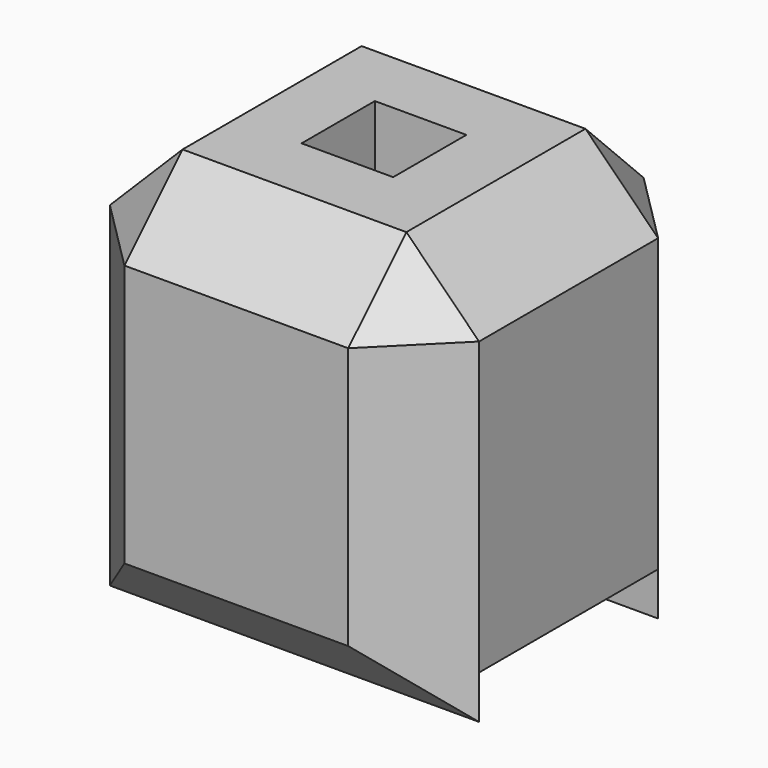
from build123d import *

# Parameters (mm, degrees)
F1_DEPTH = 2.54
F2_SIZE  = 0.49999
F3_W     = 0.63
F3_H     = 0.63
F4_DEPTH = 2.505


# Not quite as in the source:
# - a fillet or chamfer is up to 0.001 mm smaller than in the source, because OpenCascade refuses the exact size


with BuildPart() as f1:
    # F0 (on Right) → F1 (new body)
    with BuildSketch(Plane.YZ):
        Polygon((1.27, 1.402), (-1.27, 1.402), (-1.27, -1.402), (-0.77, -1.402), (-0.77, -1.103), (0.77, -1.103), (0.77, -1.402), (1.27, -1.402), align=None)
    extrude(amount=F1_DEPTH)

    # F2 (size 0.5 in the source; OpenCascade refuses exactly that, so slightly less here)
    f2_edges = [f1.edges().sort_by_distance(p)[0] for p in [
        (2.54, 0, 1.402),
        (0, 0, 1.402),
        (1.27, -1.27, 1.402),
        (1.27, 1.27, 1.402),
        (2.54, 1.27, 0),
        (1.27, 1.27, -1.402),
        (0, 1.27, 0),
        (2.54, -1.27, 0),
        (0, -1.27, 0),
        (1.27, -1.27, -1.402),
    ]]
    chamfer(f2_edges, length=F2_SIZE)

    # F3 (on face) → F4 (cut, through all)
    with BuildSketch(Plane.XY.offset(1.402)):
        with Locations((1.27, 0)):
            Rectangle(F3_W, F3_H)
    extrude(amount=-F4_DEPTH, mode=Mode.SUBTRACT)


solid = f1.part
